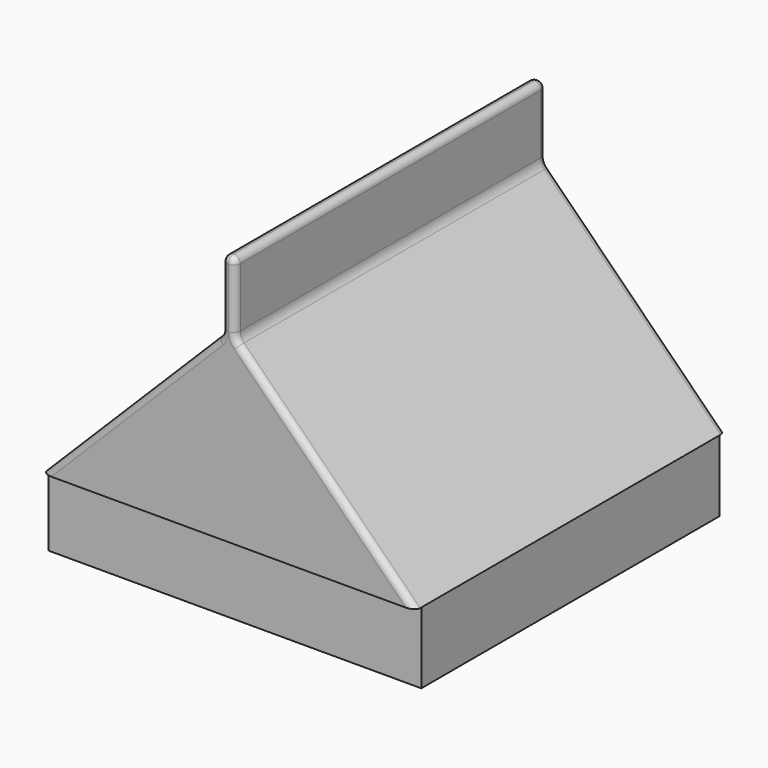
from build123d import *

# Parameters (mm, degrees)
F1_DEPTH = 38.1
F2_W     = 73.152
F2_H     = 1.524
F3_DEPTH = 13.97
F4_R     = 4.445
F5_DEPTH = 76.2
F6_R     = 33.655
F6_R_2   = 4.445
F7_DEPTH = 15.24
F8_R     = 2.54
F9_R     = 1.26999


# Not quite as in the source:
# - a fillet or chamfer is up to 0.001 mm smaller than in the source, because OpenCascade refuses the exact size


with BuildPart() as f1:
    # F0 (on Front) → F1 (new body, symmetric)
    with BuildSketch(Plane.XZ):
        Polygon((-36.576, 6.985), (-36.576, -6.985), (36.576, -6.985), (36.576, 6.985), (1.27, 42.291), (1.27, 56.261), (0, 56.261), (-1.27, 56.261), (-1.27, 42.291), align=None)
    extrude(amount=F1_DEPTH, both=True)

    # F2 (on face) → F3 (cut)
    with BuildSketch(Plane(origin=(0, 0, -6.985), x_dir=(1, 0, 0), z_dir=(0, 0, -1))):
        with Locations((0, 37.338)):
            Rectangle(F2_W, F2_H)
        with Locations((0, -37.338)):
            Rectangle(F2_W, F2_H)
    extrude(amount=-F3_DEPTH, mode=Mode.SUBTRACT)

    # F4 (on face) → F5 (cut)
    with BuildSketch(Plane(origin=(0, 0, -6.985), x_dir=(1, 0, 0), z_dir=(0, 0, -1))):
        with Locations((-12.7, 0)):
            Circle(F4_R)
    extrude(amount=-F5_DEPTH, mode=Mode.SUBTRACT)

    # F6 (on face) → F7 (cut)
    with BuildSketch(Plane(origin=(0, 0, -6.985), x_dir=(1, 0, 0), z_dir=(0, 0, -1))):
        Circle(F6_R)
        with Locations((-12.7, 0)):
            Circle(F6_R_2, mode=Mode.SUBTRACT)
    extrude(amount=-F7_DEPTH, mode=Mode.SUBTRACT)

    # F8
    f8_edges = [f1.edges().sort_by_distance(p)[0] for p in [
        (-1.27, 0, 42.291),
        (1.27, 0, 42.291),
    ]]
    fillet(f8_edges, radius=F8_R)

    # F9 (radius 1.27 in the source; OpenCascade refuses exactly that, so slightly less here)
    f9_edges = [f1.edges().sort_by_distance(p)[0] for p in [
        (-1.27, 0, 56.261),
        (0, -38.1, 56.261),
        (1.27, 0, 56.261),
        (0, 38.1, 56.261),
        (-1.27, -38.1, 49.802051),
        (19.294974, -38.1, 24.266026),
        (1.27, -38.1, 49.802051),
        (-1.27, 38.1, 49.802051),
        (1.27, 38.1, 49.802051),
    ]]
    fillet(f9_edges, radius=F9_R)


solid = f1.part
